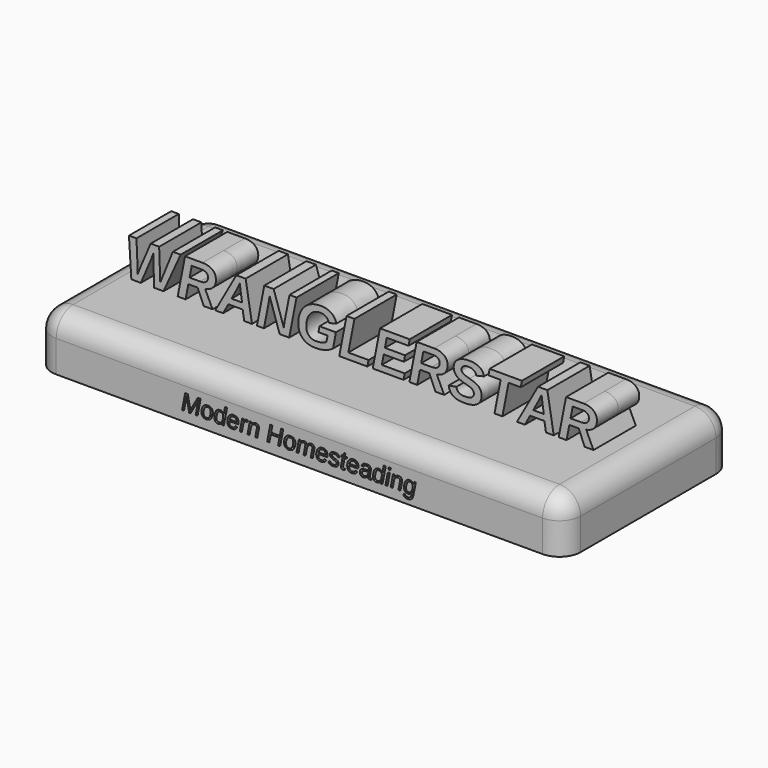
from build123d import *

# Parameters (mm, degrees)
F0_TEXT_SIZE = 13.1788783397
F2_DEPTH     = 6.35
F1_W         = 127
F1_H         = 50.8
F3_DEPTH     = 12.7
F4_R         = 5.08
F5_TEXT_SIZE = 5.5734598492
F6_DEPTH     = 1.778


# Not quite as in the source:
# - Text() gives the source's letters only with a copy of the font that has no kerning and outlines rounded to 1/6400 em; it was checked with that copy


with BuildPart() as f2:
    # F0 (on Front) → F2 (new body, symmetric)
    with BuildSketch(Plane.XZ):
        with Locations((-57.15, 0.5773799428)):
            Text('WRANGLERSTAR', F0_TEXT_SIZE, font='Arimo', font_style=FontStyle.BOLDITALIC, text_align=(TextAlign.LEFT, TextAlign.BOTTOM))
    extrude(amount=F2_DEPTH, both=True)


with BuildPart() as f3:
    # F1 (on Top) → F3 (new body)
    with BuildSketch(Plane.XY):
        Rectangle(F1_W, F1_H)
    extrude(amount=-F3_DEPTH)

    # F4
    f4_edges = [f3.edges().sort_by_distance(p)[0] for p in [
        (-63.5, -25.4, -6.35),
        (0, -25.4, 0),
        (-63.5, 0, 0),
        (-63.5, 25.4, -6.35),
        (0, 25.4, 0),
        (63.5, 0, 0),
        (63.5, -25.4, -6.35),
        (63.5, 25.4, -6.35),
    ]]
    fillet(f4_edges, radius=F4_R)

    # F5 (on face) → F6 (cut)
    with BuildSketch(Plane.XZ.offset(25.4)):
        with Locations((-28.3593312482, -10.4180714116)):
            Text('Modern Homesteading', F5_TEXT_SIZE, font='Arimo', font_style=FontStyle.ITALIC, text_align=(TextAlign.LEFT, TextAlign.BOTTOM))
    extrude(amount=-F6_DEPTH, mode=Mode.SUBTRACT)


solid = Compound([f2.part, f3.part])
